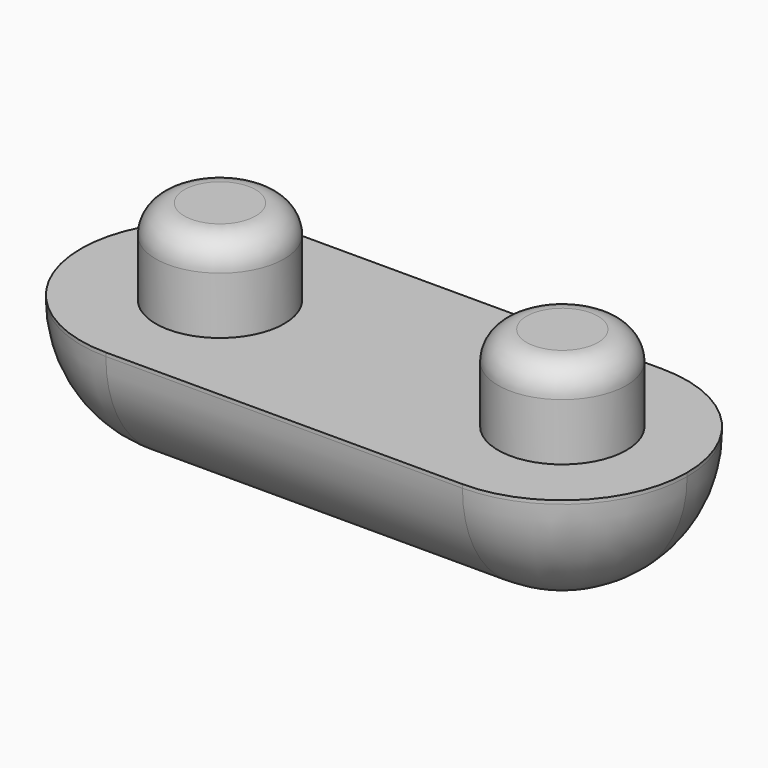
from build123d import *

# Parameters (mm, degrees)
F1_DEPTH = 9
F2_R     = 8.74999
F3_R     = 4.5
F4_DEPTH = 6
F5_R     = 2


# Not quite as in the source:
# - a fillet or chamfer is up to 0.001 mm smaller than in the source, because OpenCascade refuses the exact size


with BuildPart() as f1:
    # F0 (on Top) → F1 (new body)
    with BuildSketch(Plane.XY):
        with BuildLine():
            Line((12.5, 8.75), (-12.5, 8.75))
            ThreePointArc((-12.5, 8.75), (-18.6871843354, 6.1871843354), (-21.25, 0))
            ThreePointArc((-21.25, 0), (-18.6871843354, -6.1871843354), (-12.5, -8.75))
            Line((-12.5, -8.75), (12.5, -8.75))
            ThreePointArc((12.5, -8.75), (18.6871843354, -6.1871843354), (21.25, 0))
            ThreePointArc((21.25, 0), (18.6871843354, 6.1871843354), (12.5, 8.75))
        make_face()
    extrude(amount=F1_DEPTH)

    # F2 (radius 8.75 in the source; OpenCascade refuses exactly that, so slightly less here)
    f2_edges = [f1.edges().sort_by_distance(p)[0] for p in [
        (21.25, 0, 0),
        (-21.25, 0, 0),
        (0, -8.75, 0),
        (0, 8.75, 0),
    ]]
    fillet(f2_edges, radius=F2_R)

    # F3 (on face) → F4 (join)
    with BuildSketch(Plane.XY.offset(9)):
        with Locations((12.5, 0)):
            Circle(F3_R)
        with Locations((-11.5, 0)):
            Circle(F3_R)
    extrude(amount=F4_DEPTH)

    # F5
    f5_edges = [f1.edges().sort_by_distance(p)[0] for p in [
        (-16, 0, 15),
        (8, 0, 15),
    ]]
    fillet(f5_edges, radius=F5_R)


solid = f1.part
